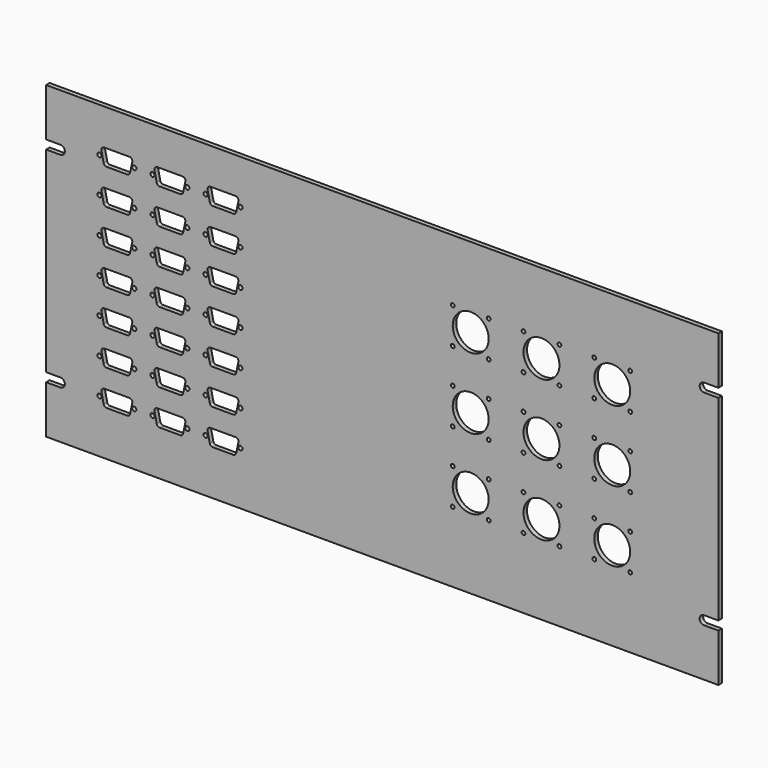
from build123d import *

# Parameters (mm, degrees)
F0_R     = 1.524
F1_DEPTH = 3.175
F2_D     = 2.7051


with BuildPart() as f1:
    # F0 (on Front) → F1 (new body)
    with BuildSketch(Plane.XZ):
        with BuildLine():
            Line((-256.0487464639, -134.9469900501), (-256.0487464639, -169.3639900501))
            Line((-256.0487464639, -169.3639900501), (226.5512535361, -169.3639900501))
            Line((226.5512535361, -169.3639900501), (226.5512535361, -134.9469900501))
            Line((226.5512535361, -134.9469900501), (216.2642535361, -134.9469900501))
            ThreePointArc((216.2642535361, -134.9469900501), (213.0892535361, -131.7719900501), (216.2642535361, -128.5969900501))
            Line((216.2642535361, -128.5969900501), (226.5512535361, -128.5969900501))
            Line((226.5512535361, -128.5969900501), (226.5512535361, 12.1190099499))
            Line((226.5512535361, 12.1190099499), (216.2642535361, 12.1190099499))
            ThreePointArc((216.2642535361, 12.1190099499), (213.0892535361, 15.2940099499), (216.2642535361, 18.4690099499))
            Line((216.2642535361, 18.4690099499), (226.5512535361, 18.4690099499))
            Line((226.5512535361, 18.4690099499), (226.5512535361, 52.8860099499))
            Line((226.5512535361, 52.8860099499), (-256.0487464639, 52.8860099499))
            Line((-256.0487464639, 52.8860099499), (-256.0487464639, 18.4690099499))
            Line((-256.0487464639, 18.4690099499), (-245.7617464639, 18.4690099499))
            ThreePointArc((-245.7617464639, 18.4690099499), (-242.5867464639, 15.2940099499), (-245.7617464639, 12.1190099499))
            Line((-245.7617464639, 12.1190099499), (-256.0487464639, 12.1190099499))
            Line((-256.0487464639, 12.1190099499), (-256.0487464639, -128.5969900501))
            Line((-256.0487464639, -128.5969900501), (-245.7617464639, -128.5969900501))
            ThreePointArc((-245.7617464639, -128.5969900501), (-242.5867464639, -131.7719900501), (-245.7617464639, -134.9469900501))
            Line((-245.7617464639, -134.9469900501), (-256.0487464639, -134.9469900501))
        make_face()
        with Locations((-217.7455464639, -131.2639900501)):
            Circle(F0_R, mode=Mode.SUBTRACT)
        with BuildLine():
            ThreePointArc((-216.3024652945, -127.9685656518), (-215.8787436507, -126.2034791177), (-214.2403464639, -125.4219900501))
            Line((-214.2403464639, -125.4219900501), (-196.2571464639, -125.4219900501))
            ThreePointArc((-196.2571464639, -125.4219900501), (-194.618749277, -126.2034791177), (-194.1950276332, -127.9685656518))
            Line((-194.1950276332, -127.9685656518), (-195.7825276332, -135.4361656518))
            ThreePointArc((-195.7825276332, -135.4361656518), (-196.5179355314, -136.6361872369), (-197.8446464639, -137.1059900501))
            Line((-197.8446464639, -137.1059900501), (-212.6528464639, -137.1059900501))
            ThreePointArc((-212.6528464639, -137.1059900501), (-213.9795573963, -136.6361872369), (-214.7149652945, -135.4361656518))
            Line((-214.7149652945, -135.4361656518), (-216.3024652945, -127.9685656518))
        make_face(mode=Mode.SUBTRACT)
        with Locations((-192.7519464639, -131.2639900501)):
            Circle(F0_R, mode=Mode.SUBTRACT)
        with Locations((-179.6455464639, -131.2639900501)):
            Circle(F0_R, mode=Mode.SUBTRACT)
        with BuildLine():
            Line((-176.6149652945, -135.4361656518), (-178.2024652945, -127.9685656518))
            ThreePointArc((-178.2024652945, -127.9685656518), (-177.7787436507, -126.2034791177), (-176.1403464639, -125.4219900501))
            Line((-176.1403464639, -125.4219900501), (-158.1571464639, -125.4219900501))
            ThreePointArc((-158.1571464639, -125.4219900501), (-156.518749277, -126.2034791177), (-156.0950276332, -127.9685656518))
            Line((-156.0950276332, -127.9685656518), (-157.6825276332, -135.4361656518))
            ThreePointArc((-157.6825276332, -135.4361656518), (-158.4179355314, -136.6361872369), (-159.7446464639, -137.1059900501))
            Line((-159.7446464639, -137.1059900501), (-174.5528464639, -137.1059900501))
            ThreePointArc((-174.5528464639, -137.1059900501), (-175.8795573963, -136.6361872369), (-176.6149652945, -135.4361656518))
        make_face(mode=Mode.SUBTRACT)
        with Locations((-154.6519464639, -131.2639900501)):
            Circle(F0_R, mode=Mode.SUBTRACT)
        with Locations((-141.5455464639, -131.2639900501)):
            Circle(F0_R, mode=Mode.SUBTRACT)
        with BuildLine():
            Line((-138.5149652945, -135.4361656518), (-140.1024652945, -127.9685656518))
            ThreePointArc((-140.1024652945, -127.9685656518), (-139.6787436507, -126.2034791177), (-138.0403464639, -125.4219900501))
            Line((-138.0403464639, -125.4219900501), (-120.0571464639, -125.4219900501))
            ThreePointArc((-120.0571464639, -125.4219900501), (-118.418749277, -126.2034791177), (-117.9950276332, -127.9685656518))
            Line((-117.9950276332, -127.9685656518), (-119.5825276332, -135.4361656518))
            ThreePointArc((-119.5825276332, -135.4361656518), (-120.3179355314, -136.6361872369), (-121.6446464639, -137.1059900501))
            Line((-121.6446464639, -137.1059900501), (-136.4528464639, -137.1059900501))
            ThreePointArc((-136.4528464639, -137.1059900501), (-137.7795573963, -136.6361872369), (-138.5149652945, -135.4361656518))
        make_face(mode=Mode.SUBTRACT)
        with Locations((-116.5519464639, -131.2639900501)):
            Circle(F0_R, mode=Mode.SUBTRACT)
        with Locations((-217.7455464639, -105.8639900501)):
            Circle(F0_R, mode=Mode.SUBTRACT)
        with BuildLine():
            Line((-214.7149652945, -110.0361656518), (-216.3024652945, -102.5685656518))
            ThreePointArc((-216.3024652945, -102.5685656518), (-215.8787436507, -100.8034791177), (-214.2403464639, -100.0219900501))
            Line((-214.2403464639, -100.0219900501), (-196.2571464639, -100.0219900501))
            ThreePointArc((-196.2571464639, -100.0219900501), (-194.618749277, -100.8034791177), (-194.1950276332, -102.5685656518))
            Line((-194.1950276332, -102.5685656518), (-195.7825276332, -110.0361656518))
            ThreePointArc((-195.7825276332, -110.0361656518), (-196.5179355314, -111.2361872369), (-197.8446464639, -111.7059900501))
            Line((-197.8446464639, -111.7059900501), (-212.6528464639, -111.7059900501))
            ThreePointArc((-212.6528464639, -111.7059900501), (-213.9795573963, -111.2361872369), (-214.7149652945, -110.0361656518))
        make_face(mode=Mode.SUBTRACT)
        with Locations((-192.7519464639, -105.8639900501)):
            Circle(F0_R, mode=Mode.SUBTRACT)
        with Locations((-179.6455464639, -105.8639900501)):
            Circle(F0_R, mode=Mode.SUBTRACT)
        with BuildLine():
            Line((-176.6149652945, -110.0361656518), (-178.2024652945, -102.5685656518))
            ThreePointArc((-178.2024652945, -102.5685656518), (-177.7787436507, -100.8034791177), (-176.1403464639, -100.0219900501))
            Line((-176.1403464639, -100.0219900501), (-158.1571464639, -100.0219900501))
            ThreePointArc((-158.1571464639, -100.0219900501), (-156.518749277, -100.8034791177), (-156.0950276332, -102.5685656518))
            Line((-156.0950276332, -102.5685656518), (-157.6825276332, -110.0361656518))
            ThreePointArc((-157.6825276332, -110.0361656518), (-158.4179355314, -111.2361872369), (-159.7446464639, -111.7059900501))
            Line((-159.7446464639, -111.7059900501), (-174.5528464639, -111.7059900501))
            ThreePointArc((-174.5528464639, -111.7059900501), (-175.8795573963, -111.2361872369), (-176.6149652945, -110.0361656518))
        make_face(mode=Mode.SUBTRACT)
        with Locations((-154.6519464639, -105.8639900501)):
            Circle(F0_R, mode=Mode.SUBTRACT)
        with Locations((-141.5455464639, -105.8639900501)):
            Circle(F0_R, mode=Mode.SUBTRACT)
        with Locations((-217.7455464639, -80.4639900501)):
            Circle(F0_R, mode=Mode.SUBTRACT)
        with BuildLine():
            Line((-214.7149652945, -84.6361656518), (-216.3024652945, -77.1685656518))
            ThreePointArc((-216.3024652945, -77.1685656518), (-215.8787436507, -75.4034791177), (-214.2403464639, -74.6219900501))
            Line((-214.2403464639, -74.6219900501), (-196.2571464639, -74.6219900501))
            ThreePointArc((-196.2571464639, -74.6219900501), (-194.618749277, -75.4034791177), (-194.1950276332, -77.1685656518))
            Line((-194.1950276332, -77.1685656518), (-195.7825276332, -84.6361656518))
            ThreePointArc((-195.7825276332, -84.6361656518), (-196.5179355314, -85.8361872369), (-197.8446464639, -86.3059900501))
            Line((-197.8446464639, -86.3059900501), (-212.6528464639, -86.3059900501))
            ThreePointArc((-212.6528464639, -86.3059900501), (-213.9795573963, -85.8361872369), (-214.7149652945, -84.6361656518))
        make_face(mode=Mode.SUBTRACT)
        with Locations((-192.7519464639, -80.4639900501)):
            Circle(F0_R, mode=Mode.SUBTRACT)
        with Locations((-179.6455464639, -80.4639900501)):
            Circle(F0_R, mode=Mode.SUBTRACT)
        with BuildLine():
            Line((-176.6149652945, -84.6361656518), (-178.2024652945, -77.1685656518))
            ThreePointArc((-178.2024652945, -77.1685656518), (-177.7787436507, -75.4034791177), (-176.1403464639, -74.6219900501))
            Line((-176.1403464639, -74.6219900501), (-158.1571464639, -74.6219900501))
            ThreePointArc((-158.1571464639, -74.6219900501), (-156.518749277, -75.4034791177), (-156.0950276332, -77.1685656518))
            Line((-156.0950276332, -77.1685656518), (-157.6825276332, -84.6361656518))
            ThreePointArc((-157.6825276332, -84.6361656518), (-158.4179355314, -85.8361872369), (-159.7446464639, -86.3059900501))
            Line((-159.7446464639, -86.3059900501), (-174.5528464639, -86.3059900501))
            ThreePointArc((-174.5528464639, -86.3059900501), (-175.8795573963, -85.8361872369), (-176.6149652945, -84.6361656518))
        make_face(mode=Mode.SUBTRACT)
        with Locations((-154.6519464639, -80.4639900501)):
            Circle(F0_R, mode=Mode.SUBTRACT)
        with Locations((-141.5455464639, -80.4639900501)):
            Circle(F0_R, mode=Mode.SUBTRACT)
        with BuildLine():
            Line((-138.5149652945, -110.0361656518), (-140.1024652945, -102.5685656518))
            ThreePointArc((-140.1024652945, -102.5685656518), (-139.6787436507, -100.8034791177), (-138.0403464639, -100.0219900501))
            Line((-138.0403464639, -100.0219900501), (-120.0571464639, -100.0219900501))
            ThreePointArc((-120.0571464639, -100.0219900501), (-118.418749277, -100.8034791177), (-117.9950276332, -102.5685656518))
            Line((-117.9950276332, -102.5685656518), (-119.5825276332, -110.0361656518))
            ThreePointArc((-119.5825276332, -110.0361656518), (-120.3179355314, -111.2361872369), (-121.6446464639, -111.7059900501))
            Line((-121.6446464639, -111.7059900501), (-136.4528464639, -111.7059900501))
            ThreePointArc((-136.4528464639, -111.7059900501), (-137.7795573963, -111.2361872369), (-138.5149652945, -110.0361656518))
        make_face(mode=Mode.SUBTRACT)
        with Locations((-116.5519464639, -105.8639900501)):
            Circle(F0_R, mode=Mode.SUBTRACT)
        with BuildLine():
            Line((-138.5149652945, -84.6361656518), (-140.1024652945, -77.1685656518))
            ThreePointArc((-140.1024652945, -77.1685656518), (-139.6787436507, -75.4034791177), (-138.0403464639, -74.6219900501))
            Line((-138.0403464639, -74.6219900501), (-120.0571464639, -74.6219900501))
            ThreePointArc((-120.0571464639, -74.6219900501), (-118.418749277, -75.4034791177), (-117.9950276332, -77.1685656518))
            Line((-117.9950276332, -77.1685656518), (-119.5825276332, -84.6361656518))
            ThreePointArc((-119.5825276332, -84.6361656518), (-120.3179355314, -85.8361872369), (-121.6446464639, -86.3059900501))
            Line((-121.6446464639, -86.3059900501), (-136.4528464639, -86.3059900501))
            ThreePointArc((-136.4528464639, -86.3059900501), (-137.7795573963, -85.8361872369), (-138.5149652945, -84.6361656518))
        make_face(mode=Mode.SUBTRACT)
        with Locations((-116.5519464639, -80.4639900501)):
            Circle(F0_R, mode=Mode.SUBTRACT)
        with BuildLine():
            ThreePointArc((48.7512535361, -118.7671900501), (35.8480535361, -105.8639900501), (48.7512535361, -92.9607900501))
            ThreePointArc((48.7512535361, -92.9607900501), (61.6544535361, -105.8639900501), (48.7512535361, -118.7671900501))
        make_face(mode=Mode.SUBTRACT)
        with BuildLine():
            ThreePointArc((99.5512535361, -118.7671900501), (86.6480535361, -105.8639900501), (99.5512535361, -92.9607900501))
            ThreePointArc((99.5512535361, -92.9607900501), (112.4544535361, -105.8639900501), (99.5512535361, -118.7671900501))
        make_face(mode=Mode.SUBTRACT)
        with BuildLine():
            ThreePointArc((150.3512535361, -118.7671900501), (137.4480535361, -105.8639900501), (150.3512535361, -92.9607900501))
            ThreePointArc((150.3512535361, -92.9607900501), (163.2544535361, -105.8639900501), (150.3512535361, -118.7671900501))
        make_face(mode=Mode.SUBTRACT)
        with Locations((-217.7455464639, -55.0639900501)):
            Circle(F0_R, mode=Mode.SUBTRACT)
        with BuildLine():
            Line((-214.7149652945, -59.2361656518), (-216.3024652945, -51.7685656518))
            ThreePointArc((-216.3024652945, -51.7685656518), (-215.8787436507, -50.0034791177), (-214.2403464639, -49.2219900501))
            Line((-214.2403464639, -49.2219900501), (-196.2571464639, -49.2219900501))
            ThreePointArc((-196.2571464639, -49.2219900501), (-194.618749277, -50.0034791177), (-194.1950276332, -51.7685656518))
            Line((-194.1950276332, -51.7685656518), (-195.7825276332, -59.2361656518))
            ThreePointArc((-195.7825276332, -59.2361656518), (-196.5179355314, -60.4361872369), (-197.8446464639, -60.9059900501))
            Line((-197.8446464639, -60.9059900501), (-212.6528464639, -60.9059900501))
            ThreePointArc((-212.6528464639, -60.9059900501), (-213.9795573963, -60.4361872369), (-214.7149652945, -59.2361656518))
        make_face(mode=Mode.SUBTRACT)
        with Locations((-192.7519464639, -55.0639900501)):
            Circle(F0_R, mode=Mode.SUBTRACT)
        with Locations((-179.6455464639, -55.0639900501)):
            Circle(F0_R, mode=Mode.SUBTRACT)
        with BuildLine():
            Line((-176.6149652945, -59.2361656518), (-178.2024652945, -51.7685656518))
            ThreePointArc((-178.2024652945, -51.7685656518), (-177.7787436507, -50.0034791177), (-176.1403464639, -49.2219900501))
            Line((-176.1403464639, -49.2219900501), (-158.1571464639, -49.2219900501))
            ThreePointArc((-158.1571464639, -49.2219900501), (-156.518749277, -50.0034791177), (-156.0950276332, -51.7685656518))
            Line((-156.0950276332, -51.7685656518), (-157.6825276332, -59.2361656518))
            ThreePointArc((-157.6825276332, -59.2361656518), (-158.4179355314, -60.4361872369), (-159.7446464639, -60.9059900501))
            Line((-159.7446464639, -60.9059900501), (-174.5528464639, -60.9059900501))
            ThreePointArc((-174.5528464639, -60.9059900501), (-175.8795573963, -60.4361872369), (-176.6149652945, -59.2361656518))
        make_face(mode=Mode.SUBTRACT)
        with Locations((-154.6519464639, -55.0639900501)):
            Circle(F0_R, mode=Mode.SUBTRACT)
        with Locations((-141.5455464639, -55.0639900501)):
            Circle(F0_R, mode=Mode.SUBTRACT)
        with Locations((-217.7455464639, -29.6639900501)):
            Circle(F0_R, mode=Mode.SUBTRACT)
        with BuildLine():
            Line((-214.7149652945, -33.8361656518), (-216.3024652945, -26.3685656518))
            ThreePointArc((-216.3024652945, -26.3685656518), (-215.8787436507, -24.6034791177), (-214.2403464639, -23.8219900501))
            Line((-214.2403464639, -23.8219900501), (-196.2571464639, -23.8219900501))
            ThreePointArc((-196.2571464639, -23.8219900501), (-194.618749277, -24.6034791177), (-194.1950276332, -26.3685656518))
            Line((-194.1950276332, -26.3685656518), (-195.7825276332, -33.8361656518))
            ThreePointArc((-195.7825276332, -33.8361656518), (-196.5179355314, -35.0361872369), (-197.8446464639, -35.5059900501))
            Line((-197.8446464639, -35.5059900501), (-212.6528464639, -35.5059900501))
            ThreePointArc((-212.6528464639, -35.5059900501), (-213.9795573963, -35.0361872369), (-214.7149652945, -33.8361656518))
        make_face(mode=Mode.SUBTRACT)
        with Locations((-217.7455464639, -4.2639900501)):
            Circle(F0_R, mode=Mode.SUBTRACT)
        with BuildLine():
            Line((-214.7149652945, -8.4361656518), (-216.3024652945, -0.9685656518))
            ThreePointArc((-216.3024652945, -0.9685656518), (-215.8787436507, 0.7965208823), (-214.2403464639, 1.5780099499))
            Line((-214.2403464639, 1.5780099499), (-196.2571464639, 1.5780099499))
            ThreePointArc((-196.2571464639, 1.5780099499), (-194.618749277, 0.7965208823), (-194.1950276332, -0.9685656518))
            Line((-194.1950276332, -0.9685656518), (-195.7825276332, -8.4361656518))
            ThreePointArc((-195.7825276332, -8.4361656518), (-196.5179355314, -9.6361872369), (-197.8446464639, -10.1059900501))
            Line((-197.8446464639, -10.1059900501), (-212.6528464639, -10.1059900501))
            ThreePointArc((-212.6528464639, -10.1059900501), (-213.9795573963, -9.6361872369), (-214.7149652945, -8.4361656518))
        make_face(mode=Mode.SUBTRACT)
        with Locations((-192.7519464639, -29.6639900501)):
            Circle(F0_R, mode=Mode.SUBTRACT)
        with Locations((-179.6455464639, -29.6639900501)):
            Circle(F0_R, mode=Mode.SUBTRACT)
        with BuildLine():
            Line((-176.6149652945, -33.8361656518), (-178.2024652945, -26.3685656518))
            ThreePointArc((-178.2024652945, -26.3685656518), (-177.7787436507, -24.6034791177), (-176.1403464639, -23.8219900501))
            Line((-176.1403464639, -23.8219900501), (-158.1571464639, -23.8219900501))
            ThreePointArc((-158.1571464639, -23.8219900501), (-156.518749277, -24.6034791177), (-156.0950276332, -26.3685656518))
            Line((-156.0950276332, -26.3685656518), (-157.6825276332, -33.8361656518))
            ThreePointArc((-157.6825276332, -33.8361656518), (-158.4179355314, -35.0361872369), (-159.7446464639, -35.5059900501))
            Line((-159.7446464639, -35.5059900501), (-174.5528464639, -35.5059900501))
            ThreePointArc((-174.5528464639, -35.5059900501), (-175.8795573963, -35.0361872369), (-176.6149652945, -33.8361656518))
        make_face(mode=Mode.SUBTRACT)
        with Locations((-154.6519464639, -29.6639900501)):
            Circle(F0_R, mode=Mode.SUBTRACT)
        with Locations((-141.5455464639, -29.6639900501)):
            Circle(F0_R, mode=Mode.SUBTRACT)
        with Locations((-192.7519464639, -4.2639900501)):
            Circle(F0_R, mode=Mode.SUBTRACT)
        with Locations((-179.6455464639, -4.2639900501)):
            Circle(F0_R, mode=Mode.SUBTRACT)
        with BuildLine():
            Line((-176.6149652945, -8.4361656518), (-178.2024652945, -0.9685656518))
            ThreePointArc((-178.2024652945, -0.9685656518), (-177.7787436507, 0.7965208823), (-176.1403464639, 1.5780099499))
            Line((-176.1403464639, 1.5780099499), (-158.1571464639, 1.5780099499))
            ThreePointArc((-158.1571464639, 1.5780099499), (-156.518749277, 0.7965208823), (-156.0950276332, -0.9685656518))
            Line((-156.0950276332, -0.9685656518), (-157.6825276332, -8.4361656518))
            ThreePointArc((-157.6825276332, -8.4361656518), (-158.4179355314, -9.6361872369), (-159.7446464639, -10.1059900501))
            Line((-159.7446464639, -10.1059900501), (-174.5528464639, -10.1059900501))
            ThreePointArc((-174.5528464639, -10.1059900501), (-175.8795573963, -9.6361872369), (-176.6149652945, -8.4361656518))
        make_face(mode=Mode.SUBTRACT)
        with Locations((-154.6519464639, -4.2639900501)):
            Circle(F0_R, mode=Mode.SUBTRACT)
        with Locations((-141.5455464639, -4.2639900501)):
            Circle(F0_R, mode=Mode.SUBTRACT)
        with BuildLine():
            Line((-138.5149652945, -59.2361656518), (-140.1024652945, -51.7685656518))
            ThreePointArc((-140.1024652945, -51.7685656518), (-139.6787436507, -50.0034791177), (-138.0403464639, -49.2219900501))
            Line((-138.0403464639, -49.2219900501), (-120.0571464639, -49.2219900501))
            ThreePointArc((-120.0571464639, -49.2219900501), (-118.418749277, -50.0034791177), (-117.9950276332, -51.7685656518))
            Line((-117.9950276332, -51.7685656518), (-119.5825276332, -59.2361656518))
            ThreePointArc((-119.5825276332, -59.2361656518), (-120.3179355314, -60.4361872369), (-121.6446464639, -60.9059900501))
            Line((-121.6446464639, -60.9059900501), (-136.4528464639, -60.9059900501))
            ThreePointArc((-136.4528464639, -60.9059900501), (-137.7795573963, -60.4361872369), (-138.5149652945, -59.2361656518))
        make_face(mode=Mode.SUBTRACT)
        with Locations((-116.5519464639, -55.0639900501)):
            Circle(F0_R, mode=Mode.SUBTRACT)
        with BuildLine():
            Line((-138.5149652945, -33.8361656518), (-140.1024652945, -26.3685656518))
            ThreePointArc((-140.1024652945, -26.3685656518), (-139.6787436507, -24.6034791177), (-138.0403464639, -23.8219900501))
            Line((-138.0403464639, -23.8219900501), (-120.0571464639, -23.8219900501))
            ThreePointArc((-120.0571464639, -23.8219900501), (-118.418749277, -24.6034791177), (-117.9950276332, -26.3685656518))
            Line((-117.9950276332, -26.3685656518), (-119.5825276332, -33.8361656518))
            ThreePointArc((-119.5825276332, -33.8361656518), (-120.3179355314, -35.0361872369), (-121.6446464639, -35.5059900501))
            Line((-121.6446464639, -35.5059900501), (-136.4528464639, -35.5059900501))
            ThreePointArc((-136.4528464639, -35.5059900501), (-137.7795573963, -35.0361872369), (-138.5149652945, -33.8361656518))
        make_face(mode=Mode.SUBTRACT)
        with Locations((-116.5519464639, -29.6639900501)):
            Circle(F0_R, mode=Mode.SUBTRACT)
        with BuildLine():
            Line((-138.5149652945, -8.4361656518), (-140.1024652945, -0.9685656518))
            ThreePointArc((-140.1024652945, -0.9685656518), (-139.6787436507, 0.7965208823), (-138.0403464639, 1.5780099499))
            Line((-138.0403464639, 1.5780099499), (-120.0571464639, 1.5780099499))
            ThreePointArc((-120.0571464639, 1.5780099499), (-118.418749277, 0.7965208823), (-117.9950276332, -0.9685656518))
            Line((-117.9950276332, -0.9685656518), (-119.5825276332, -8.4361656518))
            ThreePointArc((-119.5825276332, -8.4361656518), (-120.3179355314, -9.6361872369), (-121.6446464639, -10.1059900501))
            Line((-121.6446464639, -10.1059900501), (-136.4528464639, -10.1059900501))
            ThreePointArc((-136.4528464639, -10.1059900501), (-137.7795573963, -9.6361872369), (-138.5149652945, -8.4361656518))
        make_face(mode=Mode.SUBTRACT)
        with Locations((-116.5519464639, -4.2639900501)):
            Circle(F0_R, mode=Mode.SUBTRACT)
        with Locations((-217.7455464639, 21.1360099499)):
            Circle(F0_R, mode=Mode.SUBTRACT)
        with BuildLine():
            Line((-214.7149652945, 16.9638343482), (-216.3024652945, 24.4314343482))
            ThreePointArc((-216.3024652945, 24.4314343482), (-215.8787436507, 26.1965208823), (-214.2403464639, 26.9780099499))
            Line((-214.2403464639, 26.9780099499), (-196.2571464639, 26.9780099499))
            ThreePointArc((-196.2571464639, 26.9780099499), (-194.618749277, 26.1965208823), (-194.1950276332, 24.4314343482))
            Line((-194.1950276332, 24.4314343482), (-195.7825276332, 16.9638343482))
            ThreePointArc((-195.7825276332, 16.9638343482), (-196.5179355314, 15.7638127631), (-197.8446464639, 15.2940099499))
            Line((-197.8446464639, 15.2940099499), (-212.6528464639, 15.2940099499))
            ThreePointArc((-212.6528464639, 15.2940099499), (-213.9795573963, 15.7638127631), (-214.7149652945, 16.9638343482))
        make_face(mode=Mode.SUBTRACT)
        with Locations((-192.7519464639, 21.1360099499)):
            Circle(F0_R, mode=Mode.SUBTRACT)
        with Locations((-179.6455464639, 21.1360099499)):
            Circle(F0_R, mode=Mode.SUBTRACT)
        with BuildLine():
            Line((-176.6149652945, 16.9638343482), (-178.2024652945, 24.4314343482))
            ThreePointArc((-178.2024652945, 24.4314343482), (-177.7787436507, 26.1965208823), (-176.1403464639, 26.9780099499))
            Line((-176.1403464639, 26.9780099499), (-158.1571464639, 26.9780099499))
            ThreePointArc((-158.1571464639, 26.9780099499), (-156.518749277, 26.1965208823), (-156.0950276332, 24.4314343482))
            Line((-156.0950276332, 24.4314343482), (-157.6825276332, 16.9638343482))
            ThreePointArc((-157.6825276332, 16.9638343482), (-158.4179355314, 15.7638127631), (-159.7446464639, 15.2940099499))
            Line((-159.7446464639, 15.2940099499), (-174.5528464639, 15.2940099499))
            ThreePointArc((-174.5528464639, 15.2940099499), (-175.8795573963, 15.7638127631), (-176.6149652945, 16.9638343482))
        make_face(mode=Mode.SUBTRACT)
        with Locations((-154.6519464639, 21.1360099499)):
            Circle(F0_R, mode=Mode.SUBTRACT)
        with Locations((-141.5455464639, 21.1360099499)):
            Circle(F0_R, mode=Mode.SUBTRACT)
        with BuildLine():
            Line((-138.5149652945, 16.9638343482), (-140.1024652945, 24.4314343482))
            ThreePointArc((-140.1024652945, 24.4314343482), (-139.6787436507, 26.1965208823), (-138.0403464639, 26.9780099499))
            Line((-138.0403464639, 26.9780099499), (-120.0571464639, 26.9780099499))
            ThreePointArc((-120.0571464639, 26.9780099499), (-118.418749277, 26.1965208823), (-117.9950276332, 24.4314343482))
            Line((-117.9950276332, 24.4314343482), (-119.5825276332, 16.9638343482))
            ThreePointArc((-119.5825276332, 16.9638343482), (-120.3179355314, 15.7638127631), (-121.6446464639, 15.2940099499))
            Line((-121.6446464639, 15.2940099499), (-136.4528464639, 15.2940099499))
            ThreePointArc((-136.4528464639, 15.2940099499), (-137.7795573963, 15.7638127631), (-138.5149652945, 16.9638343482))
        make_face(mode=Mode.SUBTRACT)
        with Locations((-116.5519464639, 21.1360099499)):
            Circle(F0_R, mode=Mode.SUBTRACT)
        with BuildLine():
            ThreePointArc((48.7512535361, -67.9671900501), (35.8480535361, -55.0639900501), (48.7512535361, -42.1607900501))
            ThreePointArc((48.7512535361, -42.1607900501), (61.6544535361, -55.0639900501), (48.7512535361, -67.9671900501))
        make_face(mode=Mode.SUBTRACT)
        with BuildLine():
            ThreePointArc((99.5512535361, -67.9671900501), (86.6480535361, -55.0639900501), (99.5512535361, -42.1607900501))
            ThreePointArc((99.5512535361, -42.1607900501), (112.4544535361, -55.0639900501), (99.5512535361, -67.9671900501))
        make_face(mode=Mode.SUBTRACT)
        with BuildLine():
            ThreePointArc((48.7512535361, -17.1671900501), (35.8480535361, -4.2639900501), (48.7512535361, 8.6392099499))
            ThreePointArc((48.7512535361, 8.6392099499), (61.6544535361, -4.2639900501), (48.7512535361, -17.1671900501))
        make_face(mode=Mode.SUBTRACT)
        with BuildLine():
            ThreePointArc((99.5512535361, -17.1671900501), (86.6480535361, -4.2639900501), (99.5512535361, 8.6392099499))
            ThreePointArc((99.5512535361, 8.6392099499), (112.4544535361, -4.2639900501), (99.5512535361, -17.1671900501))
        make_face(mode=Mode.SUBTRACT)
        with BuildLine():
            ThreePointArc((150.3512535361, -67.9671900501), (137.4480535361, -55.0639900501), (150.3512535361, -42.1607900501))
            ThreePointArc((150.3512535361, -42.1607900501), (163.2544535361, -55.0639900501), (150.3512535361, -67.9671900501))
        make_face(mode=Mode.SUBTRACT)
        with BuildLine():
            ThreePointArc((150.3512535361, -17.1671900501), (137.4480535361, -4.2639900501), (150.3512535361, 8.6392099499))
            ThreePointArc((150.3512535361, 8.6392099499), (163.2544535361, -4.2639900501), (150.3512535361, -17.1671900501))
        make_face(mode=Mode.SUBTRACT)
    extrude(amount=F1_DEPTH)

    # F2 (through all)
    with Locations(Plane(origin=(0, 0, 0), x_dir=(1, 0, 0), z_dir=(0, 1, 0))):
        with Locations((35.8544035361, -8.6328599499), (61.6481035361, -8.6328599499), (61.6481035361, 17.1608400501), (35.8544035361, 17.1608400501), (86.6544035361, 17.1608400501), (112.4481035361, 17.1608400501), (112.4481035361, -8.6328599499), (86.6544035361, -8.6328599499), (35.8544035361, 42.1671400501), (61.6481035361, 42.1671400501), (86.6544035361, 42.1671400501), (112.4481035361, 42.1671400501), (137.4544035361, -8.6328599499), (163.2481035361, -8.6328599499), (163.2481035361, 17.1608400501), (137.4544035361, 17.1608400501), (137.4544035361, 42.1671400501), (163.2481035361, 42.1671400501), (35.8544035361, 67.9608400501), (61.6481035361, 67.9608400501), (86.6544035361, 67.9608400501), (112.4481035361, 67.9608400501), (137.4544035361, 67.9608400501), (163.2481035361, 67.9608400501), (163.2481035361, 92.9671400501), (137.4544035361, 92.9671400501), (112.4481035361, 92.9671400501), (86.6544035361, 92.9671400501), (61.6481035361, 92.9671400501), (35.8544035361, 92.9671400501), (35.8544035361, 118.7608400501), (61.6481035361, 118.7608400501), (86.6544035361, 118.7608400501), (112.4481035361, 118.7608400501), (137.4544035361, 118.7608400501), (163.2481035361, 118.7608400501)):
            Hole(F2_D / 2)


solid = f1.part
